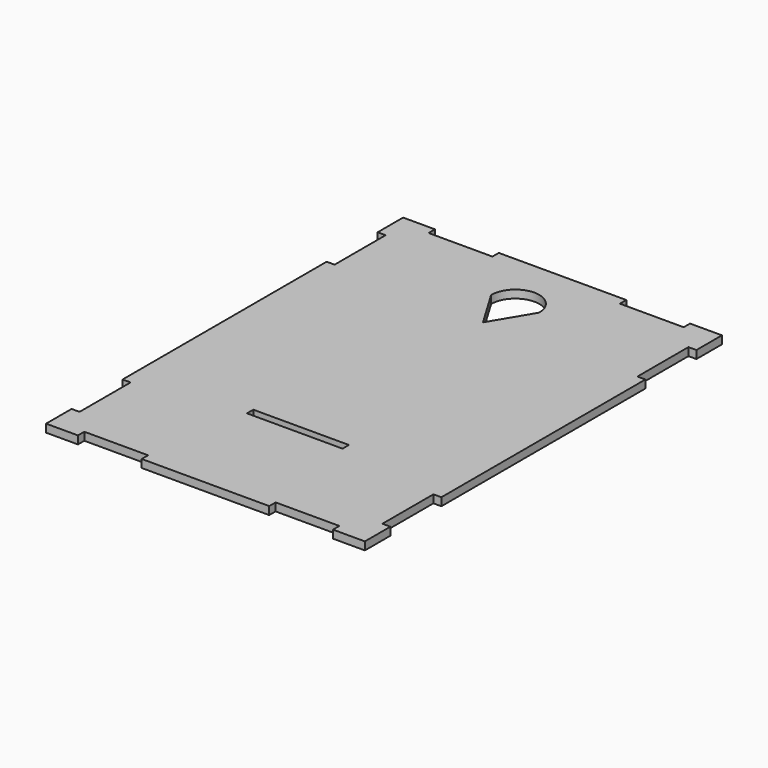
from build123d import *

# Parameters (mm, degrees)
F0_W             = 254
F0_H             = 355.6
F1_DEPTH         = 6.35
F2_W             = 50.8
F2_H             = 6.35
F3_DEPTH         = 6.351
F3_COPIES2_COUNT = 2
F3_COPIES3_COUNT = 2
F3_COPIES3_ANGLE = 90
F3_COPIES4_COUNT = 2
F3_COPIES4_ANGLE = 90
F4_W             = 6.35
F4_H             = 50.8
F5_DEPTH         = 25.4
F6_W             = 76.2
F6_H             = 6.35
F7_DEPTH         = 25.4
F9_DEPTH         = 25.4


# Not quite as in the source:
# - a pattern or mirror of a feature is missing from the dataset's text; its kind, count and spacing are read off the source's solid


with BuildPart() as f1:
    # F0 (on Top) → F1 (new body)
    with BuildSketch(Plane.XY):
        Rectangle(F0_W, F0_H)
    extrude(amount=F1_DEPTH)

    # F2 (on face) → F3 (cut, through all)
    with BuildSketch(Plane.XY.offset(6.35)):
        with Locations((-76.2, 174.625)):
            Rectangle(F2_W, F2_H)
    f3 = extrude(amount=-F3_DEPTH, mode=Mode.SUBTRACT)

    # F3_copies: F3 across plane
    add(f3.mirror(Plane(origin=(0, 0, 0), x_dir=(0, 0, -1), z_dir=(0, -1, 0))), mode=Mode.SUBTRACT)

    # F3_copies1: F3 across plane
    add(f3.mirror(Plane(origin=(0, 0, 0), x_dir=(0, 0, 1), z_dir=(1, 0, 0))), mode=Mode.SUBTRACT)

    # F3_copies2: F3 ×2 about axis
    f3_copies2_axis = Axis((0, 0, 0), (0, 0, 1))
    for i in range(1, F3_COPIES2_COUNT):
        add(f3.rotate(f3_copies2_axis, i * 360 / F3_COPIES2_COUNT), mode=Mode.SUBTRACT)

    # F3_copies3: F3 ×2 about axis
    f3_copies3_axis = Axis((50.8, 0, 0), (0, 0, 1))
    for i in range(1, F3_COPIES3_COUNT):
        add(f3.rotate(f3_copies3_axis, i * F3_COPIES3_ANGLE / (F3_COPIES3_COUNT - 1)), mode=Mode.SUBTRACT)

    # F3_copies4: F3 ×2 about axis
    f3_copies4_axis = Axis((-76.2, 127, 0), (0, 0, 1))
    for i in range(1, F3_COPIES4_COUNT):
        add(f3.rotate(f3_copies4_axis, i * F3_COPIES4_ANGLE / (F3_COPIES4_COUNT - 1)), mode=Mode.SUBTRACT)

    # F4 (on face) → F5 (cut)
    with BuildSketch(Plane.XY.offset(6.35)):
        with Locations((123.825, 127)):
            Rectangle(F4_W, F4_H)
        with Locations((123.825, -127)):
            Rectangle(F4_W, F4_H)
    extrude(amount=-F5_DEPTH, mode=Mode.SUBTRACT)

    # F6 (on face) → F7 (cut)
    with BuildSketch(Plane.XY.offset(6.35)):
        with Locations((0, -85.725)):
            Rectangle(F6_W, F6_H)
    extrude(amount=-F7_DEPTH, mode=Mode.SUBTRACT)

    # F8 (on face) → F9 (cut)
    with BuildSketch(Plane.XY.offset(6.35)):
        with BuildLine():
            Line((0, 98.5919060208), (19.05, 130.4880061596))
            ThreePointArc((19.05, 130.4880061596), (0, 149.8517760723), (-19.05, 130.4880061596))
            Line((-19.05, 130.4880061596), (0, 98.5919060208))
        make_face()
    extrude(amount=-F9_DEPTH, mode=Mode.SUBTRACT)


solid = f1.part
